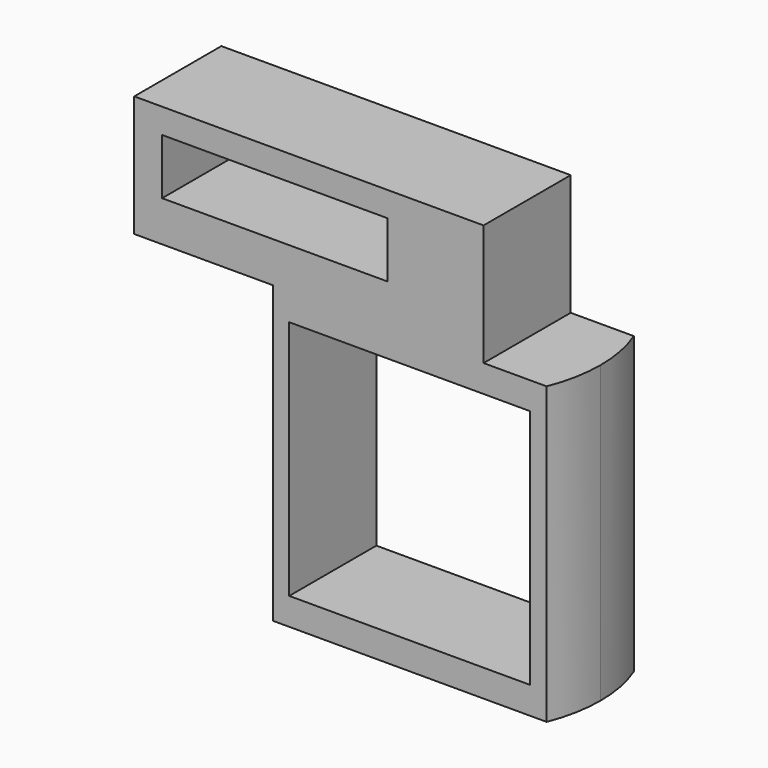
from build123d import *

# Parameters (mm, degrees)
F0_W          = 16.5766410064
F0_H          = 4.0903398767
F1_DEPTH      = 4
F1_DEPTH_BACK = 4
F3_DEPTH      = 21.7


with BuildPart() as f1:
    # F0 (on Front) → F1 (new body, two sides)
    with BuildSketch(Plane.XZ) as f1_sk:
        Polygon((-10.85, 10.85), (-10.85, 0), (-10.85, -10.85), (0, -10.85), (10.85, -10.85), (10.85, 0), (10.85, 10.85), (5.425, 10.85), (0, 10.85), align=None)
        Polygon((8.85, 8.85), (8.85, 0), (8.85, -8.85), (0, -8.85), (-8.85, -8.85), (-8.85, 0), (-8.85, 8.85), (0, 8.85), align=None, mode=Mode.SUBTRACT)
        Polygon((-20.2364195138, 10.85), (-10.85, 10.85), (0, 10.85), (5.425, 10.85), (5.425, 19.7520367801), (-20.2364195138, 19.7520367801), align=None)
        with Locations((-9.9029276753, 15.8769781701)):
            Rectangle(F0_W, F0_H, mode=Mode.SUBTRACT)
    extrude(amount=F1_DEPTH)
    extrude(f1_sk.sketch, amount=-F1_DEPTH_BACK)

    # F2 (on face) → F3 (cut)
    with BuildSketch(Plane(origin=(0, 0, -10.85), x_dir=(1, 0, 0), z_dir=(0, 0, -1))):
        with BuildLine():
            Line((13.9217844345, 4.8126999282), (9.694906495, 4.8126999282))
            ThreePointArc((9.694906495, 4.8126999282), (9.8845588749, 4.4100780486), (10.0574993187, 4))
            Line((10.0574993187, 4), (10.85, 4))
            Line((10.85, 4), (10.85, -4))
            Line((10.85, -4), (10.0574993187, -4))
            ThreePointArc((10.0574993187, -4), (9.8311449192, -4.52790041), (9.5771050518, -5.0430498086))
            Line((9.5771050518, -5.0430498086), (13.9217844345, -5.0430498086))
            Line((13.9217844345, -5.0430498086), (13.9217844345, 4.8126999282))
        make_face()
        with BuildLine():
            Line((10.85, 4), (10.0574993187, 4))
            ThreePointArc((10.0574993187, 4), (10.6304521223, 2.0363644618), (10.8237374574, 0))
            ThreePointArc((10.8237374574, 0), (10.6304521223, -2.0363644618), (10.0574993187, -4))
            Line((10.0574993187, -4), (10.85, -4))
            Line((10.85, -4), (10.85, 4))
        make_face()
        with BuildLine():
            ThreePointArc((-10.0574993187, -4), (-10.8237374574, 0), (-10.0574993187, 4))
            Line((-10.0574993187, 4), (-10.85, 4))
            Line((-10.85, 4), (-10.85, -4))
            Line((-10.85, -4), (-10.0574993187, -4))
        make_face()
    extrude(amount=-F3_DEPTH, mode=Mode.SUBTRACT)


solid = f1.part
